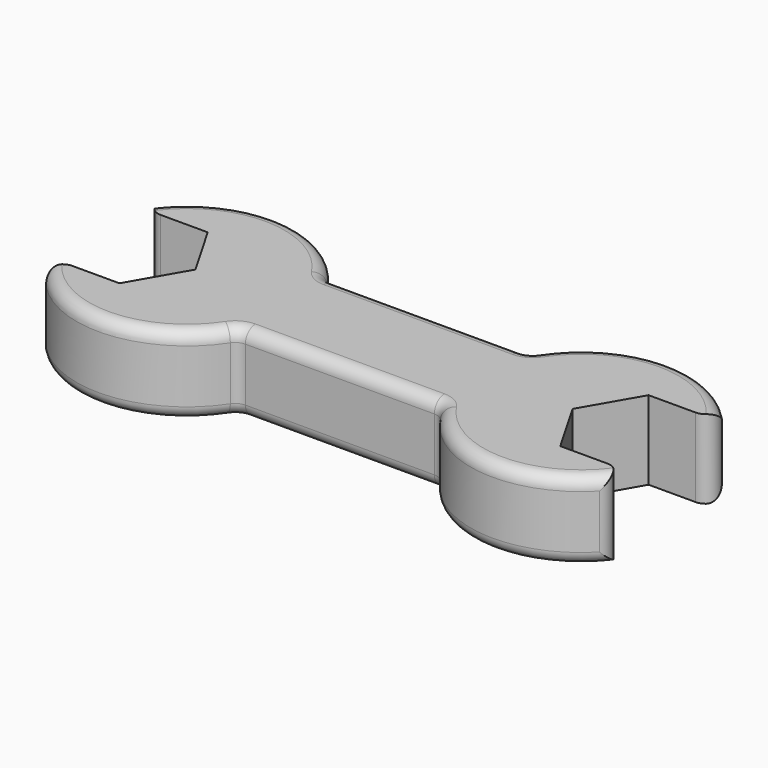
from build123d import *

# Parameters (mm, degrees)
F1_DEPTH = 6.35
F3_DEPTH = 12.701
F7_R     = 2.032


# Not quite as in the source:
# - a feature of the source that left no trace in its solid (it failed there, or was rolled back) is left out


with BuildPart() as f1:
    # F0 (on Top) → F1 (new body, symmetric)
    with BuildSketch(Plane.XY):
        with BuildLine():
            Line((16.3520683207, 8.89), (-16.3520683207, 8.89))
            ThreePointArc((-16.3520683207, 8.89), (-49.53, 0), (-16.3520683207, -8.89))
            Line((-16.3520683207, -8.89), (16.3520683207, -8.89))
            ThreePointArc((16.3520683207, -8.89), (49.53, 0), (16.3520683207, 8.89))
        make_face()
    extrude(amount=F1_DEPTH, both=True)

    # F4: F3 across plane


with BuildPart() as f3:
    # F2 (on face) → F3 (new body, through all)
    with BuildSketch(Plane.XY.offset(6.35)):
        Polygon((-35.5073561069, -8.89), (-30.3747122138, 0), (-35.5073561069, 8.89), (-45.7726438931, 8.89), (-49.53, 8.89), (-49.53, 0), (-49.53, -8.89), (-45.7726438931, -8.89), align=None)
    extrude(amount=-F3_DEPTH)


with BuildPart() as f1_1:
    add(f1.part)
    add(f3.part.mirror(Plane.YZ), mode=Mode.SUBTRACT)

    # F5: cut F3
    add(f3.part, mode=Mode.SUBTRACT)

    # F7
    f7_edges = [f1_1.edges().sort_by_distance(p)[0] for p in [
        (0, -8.89, 6.35),
        (-31.75, -17.78, 6.35),
        (-31.75, 17.78, 6.35),
        (0, 8.89, 6.35),
        (31.75, 17.78, 6.35),
        (31.75, -17.78, 6.35),
        (-31.75, -17.78, -6.35),
        (0, -8.89, -6.35),
        (31.75, -17.78, -6.35),
        (31.75, 17.78, -6.35),
        (0, 8.89, -6.35),
        (-31.75, 17.78, -6.35),
        (-16.352068, -8.89, 0),
        (16.352068, -8.89, 0),
        (-16.352068, 8.89, 0),
        (16.352068, 8.89, 0),
        (-47.147932, 8.89, 0),
        (47.147932, 8.89, 0),
        (47.147932, -8.89, 0),
        (-47.147932, -8.89, 0),
    ]]
    fillet(f7_edges, radius=F7_R)


solid = f1_1.part
